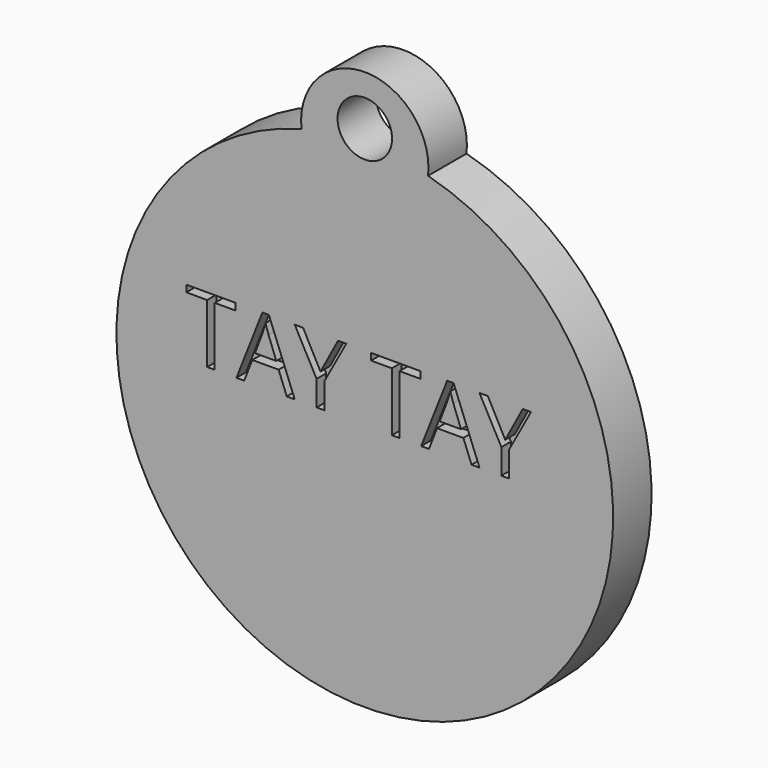
from build123d import *

# Parameters (mm, degrees)
F0_R         = 26.2498156423
F1_DEPTH     = 5.08
F2_TEXT_SIZE = 9.7335749564
F3_DEPTH     = 1.27
F4_R         = 6.7304352923
F5_DEPTH     = 5.08
F6_R         = 2.8796439162
F7_DEPTH     = 25.4


# Not quite as in the source:
# - Text() gives the source's letters only with a copy of the font that has no kerning and outlines rounded to 1/6400 em; it was checked with that copy


with BuildPart() as f1:
    # F0 (on Front) → F1 (new body)
    with BuildSketch(Plane.XZ):
        Circle(F0_R)
    extrude(amount=F1_DEPTH)

    # F2 (on face) → F3 (cut)
    with BuildSketch(Plane.XZ.offset(5.08)):
        with Locations((-18.9487877791, 0)):
            Text('TAY TAY', F2_TEXT_SIZE, font='Open Sans', text_align=(TextAlign.LEFT, TextAlign.BOTTOM))
    extrude(amount=-F3_DEPTH, mode=Mode.SUBTRACT)

    # F4 (on Front) → F5 (join)
    with BuildSketch(Plane.XZ):
        with Locations((0, 26.1346530169)):
            Circle(F4_R)
    extrude(amount=F5_DEPTH)

    # F6 (on Front) → F7 (cut)
    with BuildSketch(Plane.XZ):
        with Locations((0, 27.5946892798)):
            Circle(F6_R)
    extrude(amount=F7_DEPTH, mode=Mode.SUBTRACT)


solid = f1.part
